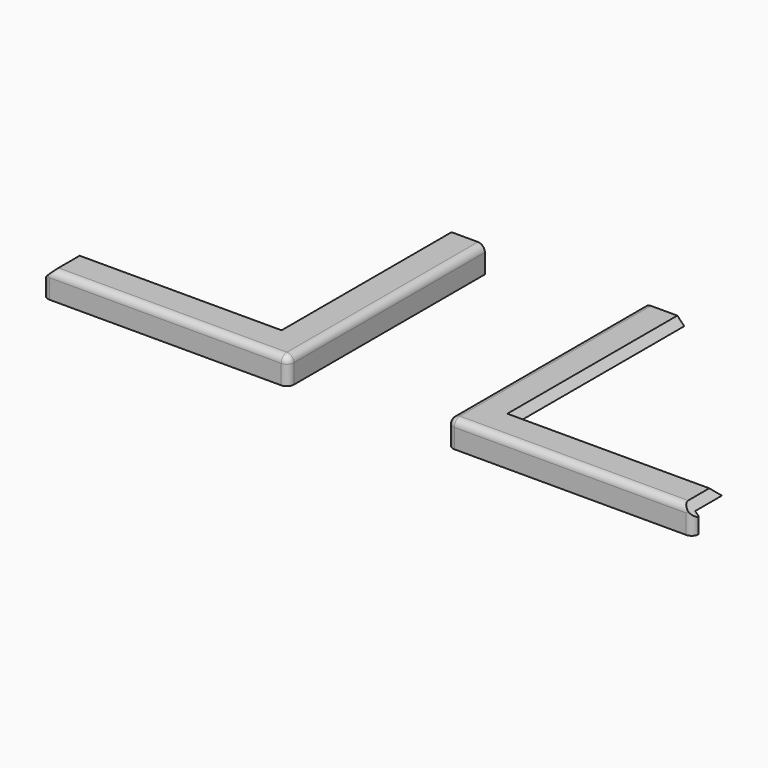
from build123d import *

# Parameters (mm, degrees)
F0_W         = 31.75
F0_H         = 146.05
F0_W_2       = 146.05
F0_H_2       = 31.75
F1_DEPTH     = 19.05
F2_T         = -5.08
F3_T1_DEPTH  = 165.6462243683
F3_T3_DEPTH  = 165.6462243683
F3_T5_DEPTH  = 70.9424487366
F3_T11_DEPTH = 185.2424487366
F3_T15_DEPTH = 185.2424487366
F4_R         = 5.08
F5_T1_DEPTH  = 26.67
F5_T3_DEPTH  = 36.83
F5_S7_W      = 5.08
F5_S7_H      = 5.08
F5_T8_DEPTH  = 5.08


# Not quite as in the source:
# - a fillet or chamfer that OpenCascade refuses, or shapes differently, is made with other operations: its cross-section is extruded or revolved along the edge and cut away or added
# - a feature names something its author has since deleted; it is built from what else it names


with BuildPart() as f1:
    # F0 (on Top) → F1 (new body)
    with BuildSketch(Plane.XY):
        with Locations((73.406, -73.025)):
            Rectangle(F0_W, F0_H)
        with Locations((162.306, -161.925)):
            Rectangle(F0_W_2, F0_H_2)
        with Locations((73.406, -161.925)):
            Rectangle(F0_W, F0_H_2)
    extrude(amount=-F1_DEPTH)

    # F2
    f2_openings = [f1.faces().sort_by_distance(p)[0] for p in [
        (86.766528, -73.025, -19.05),
        (162.306, -146.05, -9.525),
        (89.281, -73.025, -9.525),
        (73.406, 0, -9.525),
        (235.331, -161.925, -9.525),
    ]]
    offset(amount=F2_T, openings=f2_openings)

    # F3: chamfer of 7.62 on 3 edges, made by hand

    # F3_s2 → F3_t1 (cut)
    with BuildSketch(Plane.XZ.offset(-19.5962243683)):
        Polygon((81.661, 0), (89.281, -7.62), (89.281, 0), align=None)
    extrude(amount=F3_T1_DEPTH, mode=Mode.SUBTRACT)

    # F3_s4 → F3_t3 (cut)
    with BuildSketch(Plane.YZ.offset(89.281)):
        Polygon((-153.67, 0), (-146.05, -7.62), (-146.05, 0), align=None)
    extrude(amount=F3_T3_DEPTH, mode=Mode.SUBTRACT)

    # F3_s6 → F3_t5 (cut)
    with BuildSketch(Plane.XZ.offset(126.4537756317)):
        Polygon((227.711, 0), (235.331, -7.62), (235.331, 0), align=None)
    extrude(amount=F3_T5_DEPTH, mode=Mode.SUBTRACT)


with BuildPart() as f3_tool9:
    # F3_s10 → F3_t11 (new body)
    with BuildSketch(Plane.XZ.offset(165.6462243683)):
        Polygon((81.661, 0), (89.281, -7.62), (89.281, 0), align=None)
    extrude(amount=-F3_T11_DEPTH)

    split(bisect_by=Plane.XZ.offset(146.05), keep=Keep.TOP)


with BuildPart() as f3_tool13:
    # F3_s14 → F3_t15 (new body)
    with BuildSketch(Plane.YZ.offset(254.9272243683)):
        Polygon((-153.67, 0), (-146.05, -7.62), (-146.05, 0), align=None)
    extrude(amount=-F3_T15_DEPTH)

    split(bisect_by=Plane.YZ.offset(89.281), keep=Keep.BOTTOM)


with BuildPart() as f3_tool9_1:
    add(f3_tool9.part)

    # F3_t17: intersect F3_tool13
    add(f3_tool13.part, mode=Mode.INTERSECT)


with BuildPart() as f1_1:
    add(f1.part)

    # F3_t7: cut F3_tool9
    add(f3_tool9_1.part, mode=Mode.SUBTRACT)

    # F4
    f4_edges = [f1_1.edges().sort_by_distance(p)[0] for p in [
        (142.621, -177.8, 0),
        (57.531, -88.9, 0),
    ]]
    fillet(f4_edges, radius=F4_R)

    # F5: fillet of radius 5.08 on 2 edges, made by hand

    # F5_s2 → F5_t1 (cut)
    with BuildSketch(Plane.XY.offset(-31.75)):
        with BuildLine():
            ThreePointArc((57.531, -172.72), (59.0188975516, -176.3121024484), (62.611, -177.8))
            Line((62.611, -177.8), (57.531, -177.8))
            Line((57.531, -177.8), (57.531, -172.72))
        make_face()
    extrude(amount=F5_T1_DEPTH, mode=Mode.SUBTRACT)

    # F5_s4 → F5_t3 (cut)
    with BuildSketch(Plane.XY.offset(-31.75)):
        with BuildLine():
            ThreePointArc((230.251, -177.8), (233.8431024484, -176.3121024484), (235.331, -172.72))
            Line((235.331, -172.72), (235.331, -177.8))
            Line((235.331, -177.8), (230.251, -177.8))
        make_face()
    extrude(amount=F5_T3_DEPTH, mode=Mode.SUBTRACT)


with BuildPart() as f5_tool6:
    # F5_s7 → F5_t8 (new body)
    with BuildSketch(Plane.YZ.offset(62.611)):
        with Locations((-175.26, -2.54)):
            Rectangle(F5_S7_W, F5_S7_H)
    extrude(amount=-F5_T8_DEPTH)

    # F5_s9 → F5_t10 (revolve, cut)
    with BuildSketch(Plane(origin=(62.611, -172.72, -5.08), x_dir=(0, 0.7071067812, -0.7071067812), z_dir=(0, 0.7071067812, 0.7071067812))):
        with BuildLine():
            ThreePointArc((0, -5.08), (5.08, 0), (0, 5.08))
            Line((0, 5.08), (0, -5.08))
        make_face()
    revolve(axis=Axis((62.611, -172.72, -5.08), (-1, 0, 0)), mode=Mode.SUBTRACT)


with BuildPart() as f1_2:
    add(f1_1.part)

    # F5_t5: cut F5_tool6
    add(f5_tool6.part, mode=Mode.SUBTRACT)


with BuildPart() as f6_1:
    # F6: instance of F1
    add(f1_2.part.mirror(Plane.YZ))


solid = Compound([f1_2.part, f6_1.part])
